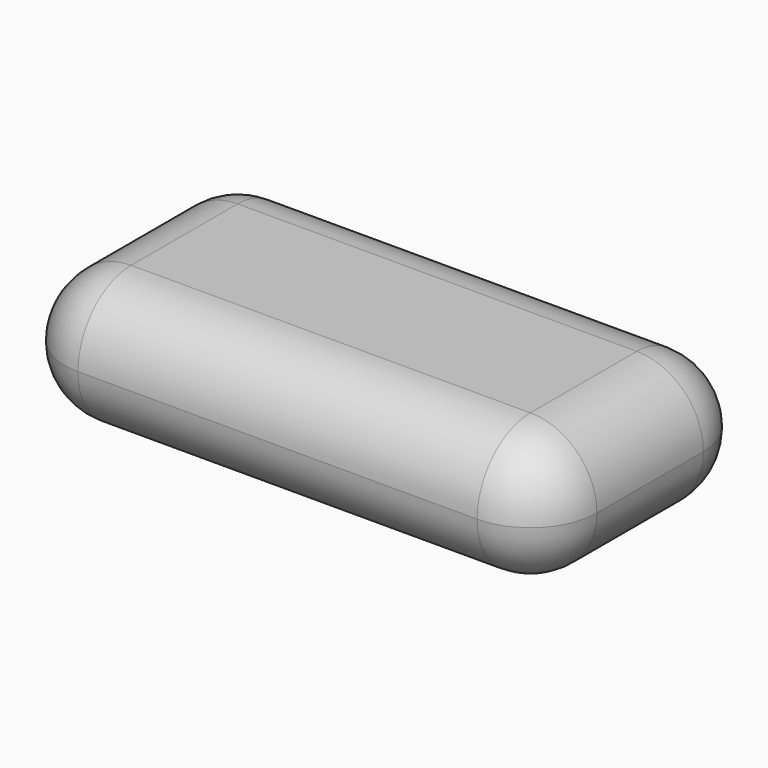
from build123d import *

# Parameters (mm, degrees)
F0_W     = 609.6
F0_H     = 304.8
F1_DEPTH = 152.4
F2_R     = 76.19999


# Not quite as in the source:
# - a fillet or chamfer is up to 0.001 mm smaller than in the source, because OpenCascade refuses the exact size


with BuildPart() as f1:
    # F0 (on Top) → F1 (new body)
    with BuildSketch(Plane.XY):
        with Locations((197.4025189088, -0.3601741046)):
            Rectangle(F0_W, F0_H)
    extrude(amount=F1_DEPTH)

    # F2 (radius 76.2 in the source; OpenCascade refuses exactly that, so slightly less here)
    f2_edges = [f1.edges().sort_by_distance(p)[0] for p in [
        (197.402519, -152.760174, 152.4),
        (-107.397481, -0.360174, 152.4),
        (197.402519, 152.039826, 152.4),
        (502.202519, -0.360174, 152.4),
        (502.202519, -152.760174, 76.2),
        (502.202519, 152.039826, 76.2),
        (502.202519, -0.360174, 0),
        (197.402519, -152.760174, 0),
        (-107.397481, -152.760174, 76.2),
        (-107.397481, -0.360174, 0),
        (-107.397481, 152.039826, 76.2),
        (197.402519, 152.039826, 0),
    ]]
    fillet(f2_edges, radius=F2_R)


solid = f1.part
